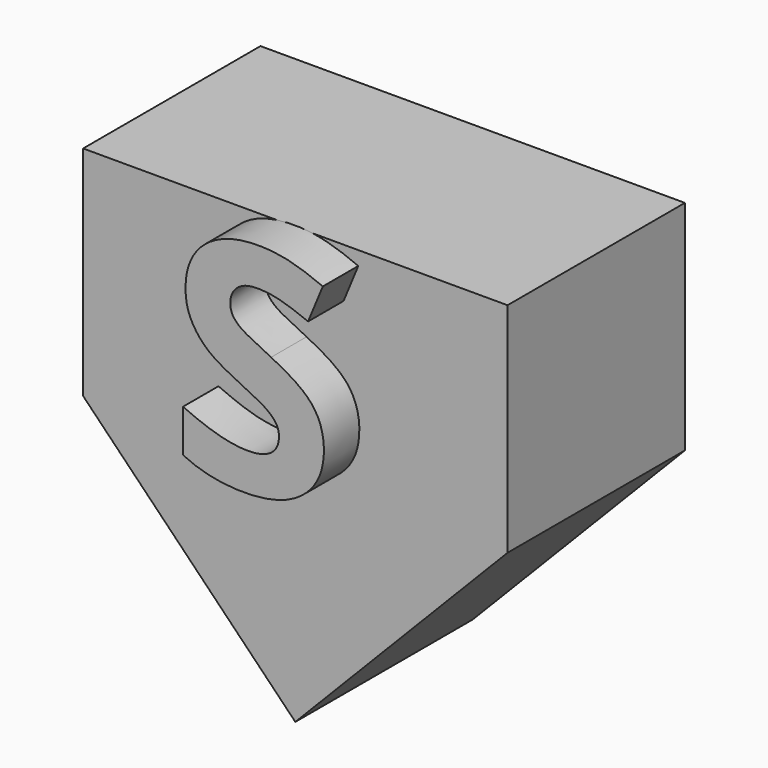
from build123d import *

# Parameters (mm, degrees)
F1_DEPTH     = 12.7
F2_TEXT_SIZE = 17.3390277778
F3_DEPTH     = 2.54


# Not quite as in the source:
# - Text() gives the source's letters only with a copy of the font that has no kerning and outlines rounded to 1/6400 em; it was checked with that copy


with BuildPart() as f1:
    # F0 (on Front) → F1 (new body)
    with BuildSketch(Plane.XZ):
        Polygon((12.1569056064, 0), (12.1569056064, 12.4841), (-12.1569056064, 12.4841), (-12.1569056064, 0), (0, -12.4841), align=None)
    extrude(amount=F1_DEPTH)

    # F2 (on face) → F3 (join)
    with BuildSketch(Plane.XZ.offset(12.7)):
        with Locations((-5.1974742673, 0)):
            Text('S', F2_TEXT_SIZE, font='Open Sans', font_style=FontStyle.BOLD, text_align=(TextAlign.LEFT, TextAlign.BOTTOM))
    extrude(amount=F3_DEPTH)


solid = f1.part
